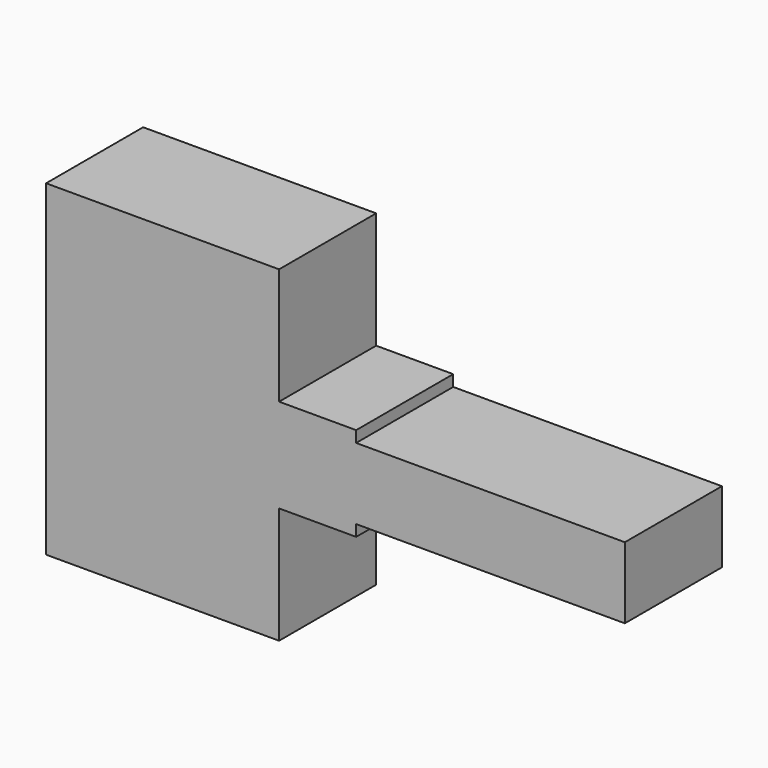
from build123d import *

# Parameters (mm, degrees)
F0_W     = 24.0008160472
F0_H     = 14.9513203651
F0_W_2   = 16.1316711456
F0_H_2   = 2.3607341573
F0_W_3   = 56.2641583383
F2_DEPTH = 12.7
F4_DEPTH = 25.4


# Not quite as in the source:
# - the program builds the solid bodies; features that only make, move or delete a surface that nothing else refers to are left out


with BuildPart() as f2:
    # F0 (on Front) → F2 (new body, symmetric)
    with BuildSketch(Plane.XZ):
        with Locations((-3.7378184497, 0)):
            Rectangle(F0_W, F0_H)
        Polygon((24.3942607194, 34.2306494713), (-24.3942607194, 34.2306494713), (-24.3942607194, -34.2306494713), (24.3942607194, -34.2306494713), (24.3942607194, -9.8363943398), (8.2625895739, -9.8363943398), (8.2625895739, -7.4756601825), (-15.7382264733, -7.4756601825), (-15.7382264733, 7.4756601825), (8.2625895739, 7.4756601825), (8.2625895739, 9.8363943398), (24.3942607194, 9.8363943398), align=None)
        with Locations((32.4600962922, 0)):
            Rectangle(F0_W_2, F0_H)
        with Locations((16.3284251466, 0)):
            Rectangle(F0_W_2, F0_H)
        with Locations((16.3284251466, 8.6560272612)):
            Rectangle(F0_W_2, F0_H_2)
        with Locations((32.4600962922, 8.6560272612)):
            Rectangle(F0_W_2, F0_H_2)
        with Locations((16.3284251466, -8.6560272612)):
            Rectangle(F0_W_2, F0_H_2)
        with Locations((32.4600962922, -8.6560272612)):
            Rectangle(F0_W_2, F0_H_2)
        with Locations((68.6580110341, 0)):
            Rectangle(F0_W_3, F0_H)
    extrude(amount=F2_DEPTH, both=True)

    # F4 (add): a face of the model
    f4_faces = [f2.faces().sort_by_distance(p)[0] for p in [
        (15.1283797196, 12.7, 0),
    ]]
    extrude(f4_faces, amount=-F4_DEPTH)


solid = f2.part
